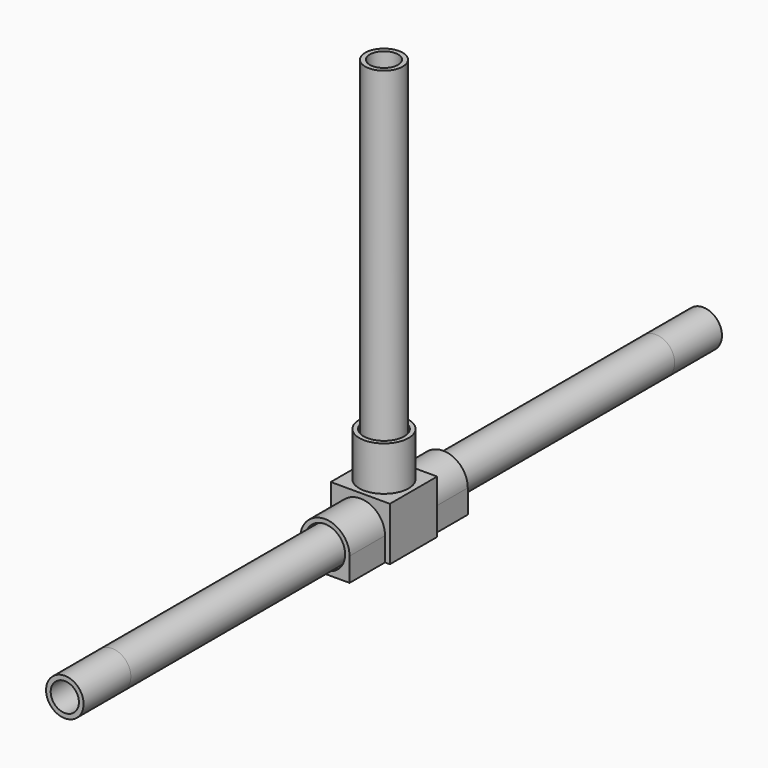
from build123d import *

# Parameters (mm, degrees)
F0_W      = 40
F0_H      = 40
F0_R      = 16.7
F0_R_2    = 13.7
F1_DEPTH  = 20
F0_R_3    = 12.7
F0_R_4    = 9.55
F2_R      = 16.7
F2_R_2    = 13.7
F3_R      = 16.7
F3_R_2    = 13.7
F4_DEPTH  = 30
F5_DEPTH  = 250
F6_R      = 13.7
F6_R_2    = 12.7
F6_R_3    = 9.55
F7_DEPTH  = 3
F8_DEPTH  = 250
F6_R_4    = 16.7
F9_DEPTH  = 30
F10_DEPTH = 3
F13_DEPTH = 30
F14_DEPTH = 30
F15_DEPTH = 4


# Not quite as in the source:
# - after a boolean that leaves OpenCascade's solid faulty, fix() repairs it


with BuildPart() as f1:
    # F0 (on Front) → F1 (new body, symmetric)
    with BuildSketch(Plane.XZ):
        Rectangle(F0_W, F0_H)
        Circle(F0_R, mode=Mode.SUBTRACT)
        Circle(F0_R)
        Circle(F0_R_2, mode=Mode.SUBTRACT)
    extrude(amount=F1_DEPTH, both=True)

    # F2 (on face) + F3 (on face) → F4 (join, symmetric)
    with BuildSketch(Plane.XZ.offset(20)):
        Circle(F2_R)
        Circle(F2_R_2, mode=Mode.SUBTRACT)
    with BuildSketch(Plane(origin=(0, 20, 0), x_dir=(-1, 0, 0), z_dir=(0, 1, 0))):
        Circle(F3_R)
        Circle(F3_R_2, mode=Mode.SUBTRACT)
    extrude(amount=F4_DEPTH, both=True, dir=(0, -1, 0))

    add(f1.part.fix(), mode=Mode.REPLACE)

    # F6 (on face) → F7 (cut)
    with BuildSketch(Plane.XY.offset(20)):
        Circle(F6_R)
        Circle(F6_R_2, mode=Mode.SUBTRACT)
        Circle(F6_R_2)
        Circle(F6_R_3, mode=Mode.SUBTRACT)
        Circle(F6_R_3)
    extrude(amount=-F7_DEPTH, mode=Mode.SUBTRACT)

    # F6 (on face) → F9 (join)
    with BuildSketch(Plane.XY.offset(20)):
        Circle(F6_R_4)
        Circle(F6_R, mode=Mode.SUBTRACT)
    extrude(amount=F9_DEPTH)

    # F11 (on face) → F13 (join, through all)
    with BuildSketch(Plane.XZ.offset(50)):
        with BuildLine():
            ThreePointArc((16.7, 0), (0, -16.7), (-16.7, 0))
            Line((-16.7, 0), (-16.7, -20))
            Line((-16.7, -20), (16.7, -20))
            Line((16.7, -20), (16.7, 0))
        make_face()
    extrude(amount=-F13_DEPTH)

    # F12 (on face) → F14 (join, through all)
    with BuildSketch(Plane(origin=(0, 50, 0), x_dir=(-1, 0, 0), z_dir=(0, 1, 0))):
        with BuildLine():
            ThreePointArc((16.7, 0), (0, -16.7), (-16.7, 0))
            Line((-16.7, 0), (-16.7, -20))
            Line((-16.7, -20), (16.7, -20))
            Line((16.7, -20), (16.7, 0))
        make_face()
    extrude(amount=-F14_DEPTH)

    # F15 (cut): a face of the model
    f15_faces = [f1.faces().sort_by_distance(p)[0] for p in [
        (0, 0, -20),
    ]]
    extrude(f15_faces, amount=-F15_DEPTH, mode=Mode.SUBTRACT)


with BuildPart() as f1b:
    # F0 (on Front) → F1, piece 2 (new body, symmetric)
    with BuildSketch(Plane.XZ):
        Circle(F0_R_3)
        Circle(F0_R_4, mode=Mode.SUBTRACT)
    extrude(amount=F1_DEPTH, both=True)

    # F5 (add, symmetric): faces of the model
    f5_faces = [f1b.faces().sort_by_distance(p)[0] for p in [
        (-12.3407897552, -20, 0),
        (-12.3407897552, 20, 0),
    ]]
    extrude(f5_faces, amount=F5_DEPTH, both=True, dir=(0, -1, 0))


with BuildPart() as f8:
    # F6 (on face) → F8 (new body)
    with BuildSketch(Plane.XY.offset(20)):
        Circle(F6_R_2)
        Circle(F6_R_3, mode=Mode.SUBTRACT)
    extrude(amount=F8_DEPTH)


with BuildPart() as f10:
    # F6 (on face) → F10 (new body)
    with BuildSketch(Plane.XY.offset(20)):
        Circle(F6_R_2)
        Circle(F6_R_3, mode=Mode.SUBTRACT)
    extrude(amount=-F10_DEPTH)


solid = Compound([f1.part, f1b.part, f8.part, f10.part])
